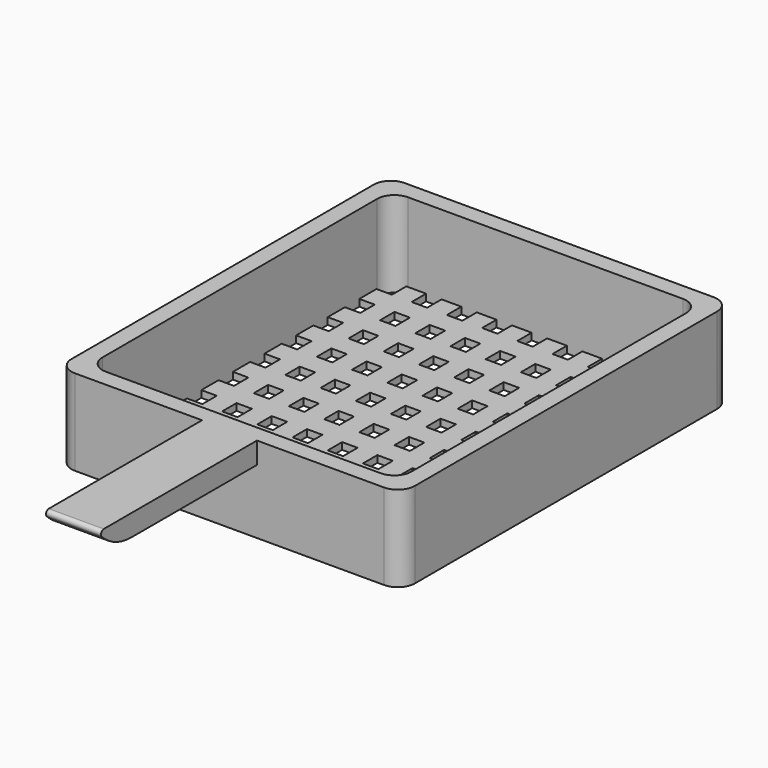
from build123d import *

# Parameters (mm, degrees)
F0_W        = 100
F0_H        = 120
F1_DEPTH    = 25
F2_W        = 90
F2_H        = 110
F3_DEPTH    = 23
F4_W        = 4.5
F4_H        = 5.25
F5_DEPTH    = 25
F6_R        = 5
F7_W        = 16
F7_H        = 6.25
F8_DEPTH    = 57.9
F9_T1_DEPTH = 76.9174646551
F10_R       = 1


# Not quite as in the source:
# - a fillet or chamfer that OpenCascade refuses, or shapes differently, is made with other operations: its cross-section is extruded or revolved along the edge and cut away or added


with BuildPart() as f1:
    # F0 (on Top) → F1 (new body)
    with BuildSketch(Plane.XY):
        Rectangle(F0_W, F0_H)
    extrude(amount=F1_DEPTH)

    # F2 (on face) → F3 (cut)
    with BuildSketch(Plane.XY.offset(25)):
        Rectangle(F2_W, F2_H)
    extrude(amount=-F3_DEPTH, mode=Mode.SUBTRACT)

    # F4 (on face) → F5 (cut)
    with BuildSketch(Plane.XY.offset(2)):
        with Locations((-42.75, 52.375)):
            Rectangle(F4_W, F4_H)
        with Locations((-42.75, 40.875)):
            Rectangle(F4_W, F4_H)
        with Locations((-42.75, 29.375)):
            Rectangle(F4_W, F4_H)
        with Locations((-42.75, 17.875)):
            Rectangle(F4_W, F4_H)
        with Locations((-42.75, 6.375)):
            Rectangle(F4_W, F4_H)
        with Locations((-42.75, -5.125)):
            Rectangle(F4_W, F4_H)
        with Locations((-42.75, -16.625)):
            Rectangle(F4_W, F4_H)
        with Locations((-42.75, -28.125)):
            Rectangle(F4_W, F4_H)
        with Locations((-42.75, -39.625)):
            Rectangle(F4_W, F4_H)
        with Locations((-42.75, -51.125)):
            Rectangle(F4_W, F4_H)
        with Locations((-32.5, 52.375)):
            Rectangle(F4_W, F4_H)
        with Locations((-32.5, 40.875)):
            Rectangle(F4_W, F4_H)
        with Locations((-32.5, 29.375)):
            Rectangle(F4_W, F4_H)
        with Locations((-32.5, 17.875)):
            Rectangle(F4_W, F4_H)
        with Locations((-32.5, 6.375)):
            Rectangle(F4_W, F4_H)
        with Locations((-32.5, -5.125)):
            Rectangle(F4_W, F4_H)
        with Locations((-32.5, -16.625)):
            Rectangle(F4_W, F4_H)
        with Locations((-32.5, -28.125)):
            Rectangle(F4_W, F4_H)
        with Locations((-32.5, -39.625)):
            Rectangle(F4_W, F4_H)
        with Locations((-32.5, -51.125)):
            Rectangle(F4_W, F4_H)
        with Locations((-22.25, 52.375)):
            Rectangle(F4_W, F4_H)
        with Locations((-22.25, 40.875)):
            Rectangle(F4_W, F4_H)
        with Locations((-22.25, 29.375)):
            Rectangle(F4_W, F4_H)
        with Locations((-22.25, 17.875)):
            Rectangle(F4_W, F4_H)
        with Locations((-22.25, 6.375)):
            Rectangle(F4_W, F4_H)
        with Locations((-22.25, -5.125)):
            Rectangle(F4_W, F4_H)
        with Locations((-22.25, -16.625)):
            Rectangle(F4_W, F4_H)
        with Locations((-22.25, -28.125)):
            Rectangle(F4_W, F4_H)
        with Locations((-22.25, -39.625)):
            Rectangle(F4_W, F4_H)
        with Locations((-22.25, -51.125)):
            Rectangle(F4_W, F4_H)
        with Locations((-12, 52.375)):
            Rectangle(F4_W, F4_H)
        with Locations((-12, 40.875)):
            Rectangle(F4_W, F4_H)
        with Locations((-12, 29.375)):
            Rectangle(F4_W, F4_H)
        with Locations((-12, 17.875)):
            Rectangle(F4_W, F4_H)
        with Locations((-12, 6.375)):
            Rectangle(F4_W, F4_H)
        with Locations((-12, -5.125)):
            Rectangle(F4_W, F4_H)
        with Locations((-12, -16.625)):
            Rectangle(F4_W, F4_H)
        with Locations((-12, -28.125)):
            Rectangle(F4_W, F4_H)
        with Locations((-12, -39.625)):
            Rectangle(F4_W, F4_H)
        with Locations((-12, -51.125)):
            Rectangle(F4_W, F4_H)
        with Locations((-1.75, 52.375)):
            Rectangle(F4_W, F4_H)
        with Locations((-1.75, 40.875)):
            Rectangle(F4_W, F4_H)
        with Locations((-1.75, 29.375)):
            Rectangle(F4_W, F4_H)
        with Locations((-1.75, 17.875)):
            Rectangle(F4_W, F4_H)
        with Locations((-1.75, 6.375)):
            Rectangle(F4_W, F4_H)
        with Locations((-1.75, -5.125)):
            Rectangle(F4_W, F4_H)
        with Locations((-1.75, -16.625)):
            Rectangle(F4_W, F4_H)
        with Locations((-1.75, -28.125)):
            Rectangle(F4_W, F4_H)
        with Locations((-1.75, -39.625)):
            Rectangle(F4_W, F4_H)
        with Locations((-1.75, -51.125)):
            Rectangle(F4_W, F4_H)
        with Locations((8.5, 52.375)):
            Rectangle(F4_W, F4_H)
        with Locations((8.5, 40.875)):
            Rectangle(F4_W, F4_H)
        with Locations((8.5, 29.375)):
            Rectangle(F4_W, F4_H)
        with Locations((8.5, 17.875)):
            Rectangle(F4_W, F4_H)
        with Locations((8.5, 6.375)):
            Rectangle(F4_W, F4_H)
        with Locations((8.5, -5.125)):
            Rectangle(F4_W, F4_H)
        with Locations((8.5, -16.625)):
            Rectangle(F4_W, F4_H)
        with Locations((8.5, -28.125)):
            Rectangle(F4_W, F4_H)
        with Locations((8.5, -39.625)):
            Rectangle(F4_W, F4_H)
        with Locations((8.5, -51.125)):
            Rectangle(F4_W, F4_H)
        with Locations((18.75, 52.375)):
            Rectangle(F4_W, F4_H)
        with Locations((18.75, 40.875)):
            Rectangle(F4_W, F4_H)
        with Locations((18.75, 29.375)):
            Rectangle(F4_W, F4_H)
        with Locations((18.75, 17.875)):
            Rectangle(F4_W, F4_H)
        with Locations((18.75, 6.375)):
            Rectangle(F4_W, F4_H)
        with Locations((18.75, -5.125)):
            Rectangle(F4_W, F4_H)
        with Locations((18.75, -16.625)):
            Rectangle(F4_W, F4_H)
        with Locations((18.75, -28.125)):
            Rectangle(F4_W, F4_H)
        with Locations((18.75, -39.625)):
            Rectangle(F4_W, F4_H)
        with Locations((18.75, -51.125)):
            Rectangle(F4_W, F4_H)
        with Locations((29, 52.375)):
            Rectangle(F4_W, F4_H)
        with Locations((29, 40.875)):
            Rectangle(F4_W, F4_H)
        with Locations((29, 29.375)):
            Rectangle(F4_W, F4_H)
        with Locations((29, 17.875)):
            Rectangle(F4_W, F4_H)
        with Locations((29, 6.375)):
            Rectangle(F4_W, F4_H)
        with Locations((29, -5.125)):
            Rectangle(F4_W, F4_H)
        with Locations((29, -16.625)):
            Rectangle(F4_W, F4_H)
        with Locations((29, -28.125)):
            Rectangle(F4_W, F4_H)
        with Locations((29, -39.625)):
            Rectangle(F4_W, F4_H)
        with Locations((29, -51.125)):
            Rectangle(F4_W, F4_H)
        with Locations((39.25, 52.375)):
            Rectangle(F4_W, F4_H)
        with Locations((39.25, 40.875)):
            Rectangle(F4_W, F4_H)
        with Locations((39.25, 29.375)):
            Rectangle(F4_W, F4_H)
        with Locations((39.25, 17.875)):
            Rectangle(F4_W, F4_H)
        with Locations((39.25, 6.375)):
            Rectangle(F4_W, F4_H)
        with Locations((39.25, -5.125)):
            Rectangle(F4_W, F4_H)
        with Locations((39.25, -16.625)):
            Rectangle(F4_W, F4_H)
        with Locations((39.25, -28.125)):
            Rectangle(F4_W, F4_H)
        with Locations((39.25, -39.625)):
            Rectangle(F4_W, F4_H)
        with Locations((39.25, -51.125)):
            Rectangle(F4_W, F4_H)
    extrude(amount=-F5_DEPTH, mode=Mode.SUBTRACT)

    # F6
    f6_edges = [f1.edges().sort_by_distance(p)[0] for p in [
        (-45, -55, 13.5),
        (-45, 55, 12.5),
        (50, -60, 12.5),
        (-50, -60, 12.5),
        (45, -55, 13.5),
        (45, 55, 13.5),
        (-50, 60, 12.5),
        (50, 60, 12.5),
    ]]
    fillet(f6_edges, radius=F6_R)

    # F7 (on face) → F8 (join)
    with BuildSketch(Plane.XZ.offset(60)):
        with Locations((0, 21.875)):
            Rectangle(F7_W, F7_H)
    extrude(amount=F8_DEPTH)

    # F9: fillet of radius 15 on 1 edges, made by hand

    # F9_s2 → F9_t1 (cut)
    with BuildSketch(Plane.YZ.offset(-38.4587323275)):
        with BuildLine():
            ThreePointArc((-105.716507069, 18.75), (-112.5630390378, 20.403652185), (-117.9, 25))
            Line((-117.9, 25), (-117.9, 18.75))
            Line((-117.9, 18.75), (-105.716507069, 18.75))
        make_face()
    extrude(amount=F9_T1_DEPTH, mode=Mode.SUBTRACT)

    # F10
    f10_edges = [f1.edges().sort_by_distance(p)[0] for p in [
        (0, -117.9, 25),
    ]]
    fillet(f10_edges, radius=F10_R)


solid = f1.part
